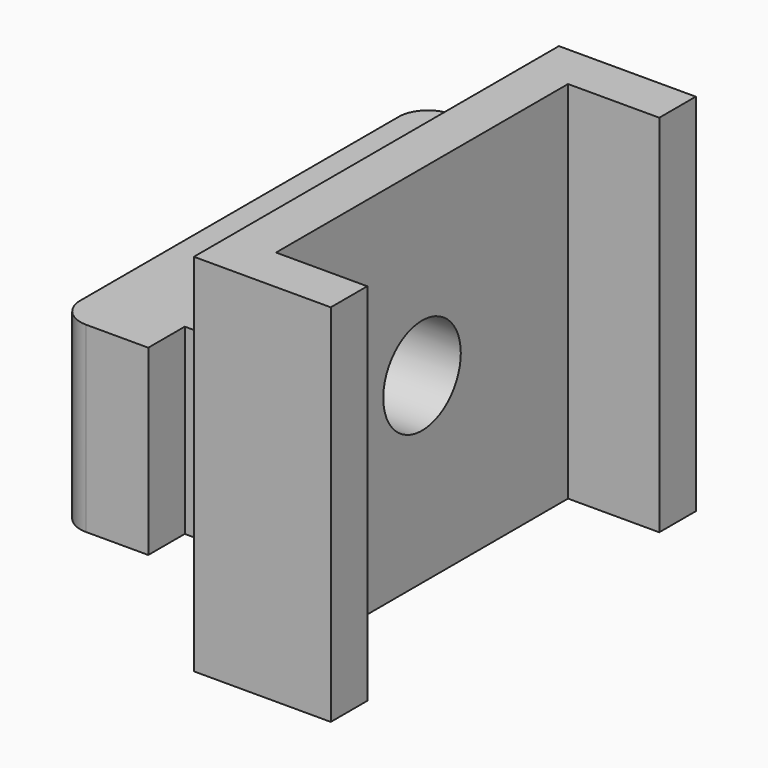
from build123d import *

# Parameters (mm, degrees)
F0_W     = 3.175
F0_H     = 6.6040001805
F0_H_2   = 3.81
F0_H_3   = 6.0959998195
F0_H_4   = 5.08
F1_DEPTH = 9.525
F0_R     = 3.3734375
F2_DEPTH = 9.525
F0_W_2   = 25.4
F3_DEPTH = 3.175
F4_START = -3.175
F4_DEPTH = 6.35
F5_R     = 2.032


# Not quite as in the source:
# - a feature names something its author has since deleted; it is built from what else it names


with BuildPart() as f1:
    # F0 (on Right) → F1 (new body)
    with BuildSketch(Plane.YZ):
        with Locations((23.2162721504, -5.0538677492)):
            Rectangle(F0_W, F0_H)
        with Locations((23.2162721504, -10.2608678395)):
            Rectangle(F0_W, F0_H_2)
        with Locations((23.2162721504, -19.1508678395)):
            Rectangle(F0_W, F0_H_2)
        with Locations((23.2162721504, -24.1038677492)):
            Rectangle(F0_W, F0_H_3)
        with Locations((23.2162721504, -14.7058678395)):
            Rectangle(F0_W, F0_H_4)
    extrude(amount=F1_DEPTH)



with BuildPart() as f1b:
    # F0 (on Right) → F1, piece 2 (new body)
    with BuildSketch(Plane.YZ):
        with Locations((-5.3587278496, -24.1038677492)):
            Rectangle(F0_W, F0_H_3)
        with Locations((-5.3587278496, -14.7058678395)):
            Rectangle(F0_W, F0_H_4)
        with Locations((-5.3587278496, -10.2608678395)):
            Rectangle(F0_W, F0_H_2)
        with Locations((-5.3587278496, -5.0538677492)):
            Rectangle(F0_W, F0_H)
        with Locations((-5.3587278496, -19.1508678395)):
            Rectangle(F0_W, F0_H_2)
    extrude(amount=F1_DEPTH)


with BuildPart() as f1_1:
    add(f1.part)

    add(f1b.part)  # F2 merges F1b
    # F0 (on Right) → F2 (join)
    with BuildSketch(Plane.YZ):
        Polygon((21.6287721504, -8.3558678395), (-3.7712278496, -8.3558678395), (-3.7712278496, -12.1658678395), (-3.7712278496, -17.2458678395), (-3.7712278496, -21.0558678395), (21.6287721504, -21.0558678395), (21.6287721504, -17.2458678395), (21.6287721504, -12.1658678395), align=None)
        with Locations((8.9287721504, -14.451867659)):
            Circle(F0_R, mode=Mode.SUBTRACT)
    extrude(amount=-F2_DEPTH)

    # F0 (on Right) → F3 (join)
    with BuildSketch(Plane.YZ):
        with Locations((8.9287721504, -5.0538677492)):
            Rectangle(F0_W_2, F0_H)
        Polygon((21.6287721504, -8.3558678395), (-3.7712278496, -8.3558678395), (-3.7712278496, -12.1658678395), (-3.7712278496, -17.2458678395), (-3.7712278496, -21.0558678395), (21.6287721504, -21.0558678395), (21.6287721504, -17.2458678395), (21.6287721504, -12.1658678395), align=None)
        with Locations((8.9287721504, -14.451867659)):
            Circle(F0_R, mode=Mode.SUBTRACT)
        with Locations((8.9287721504, -24.1038677492)):
            Rectangle(F0_W_2, F0_H_3)
    extrude(amount=F3_DEPTH)

    # F0 (on Right) → F4 (join)
    with BuildSketch(Plane.YZ.offset(F4_START)):
        with Locations((-5.3587278496, -14.7058678395)):
            Rectangle(F0_W, F0_H_4)
        with Locations((23.2162721504, -14.7058678395)):
            Rectangle(F0_W, F0_H_4)
        with Locations((23.2162721504, -19.1508678395)):
            Rectangle(F0_W, F0_H_2)
        with Locations((23.2162721504, -10.2608678395)):
            Rectangle(F0_W, F0_H_2)
        with Locations((-5.3587278496, -19.1508678395)):
            Rectangle(F0_W, F0_H_2)
        with Locations((-5.3587278496, -10.2608678395)):
            Rectangle(F0_W, F0_H_2)
    extrude(amount=-F4_DEPTH)

    # F5
    f5_edges = [f1_1.edges().sort_by_distance(p)[0] for p in [
        (-9.525, -6.946228, -14.705868),
        (-9.525, 24.803772, -14.705868),
    ]]
    fillet(f5_edges, radius=F5_R)


solid = f1_1.part
